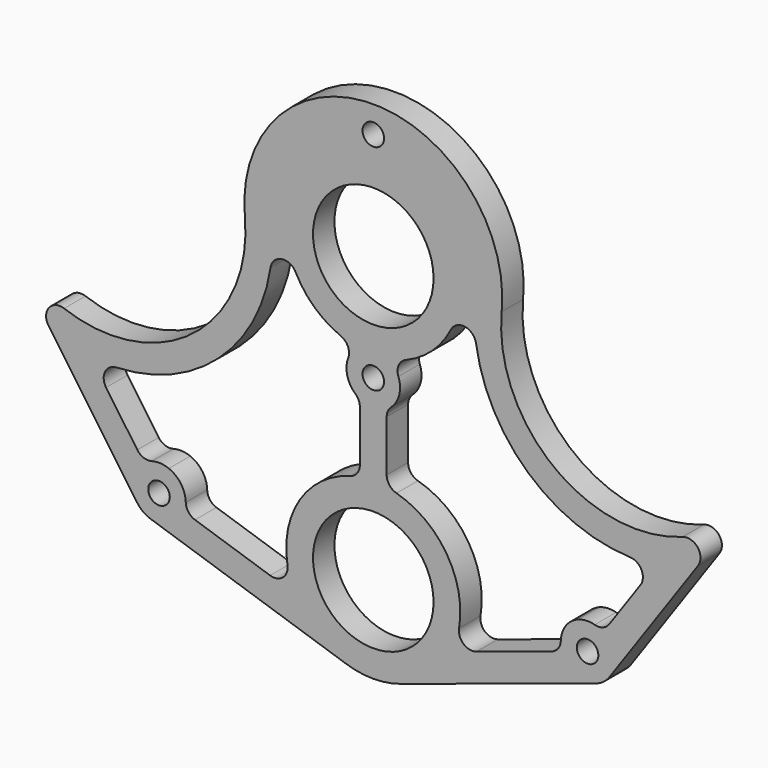
from build123d import *

# Parameters (mm, degrees)
F0_R     = 2.5527
F0_R_2   = 14.2875
F1_DEPTH = 6.35
F2_F1_R  = 3.175
F2_F2_R  = 3.175
F4_DEPTH = 25.4
F5_R     = 3.175


# Not quite as in the source:
# - a pattern or mirror of a feature is missing from the dataset's text; its kind, count and spacing are read off the source's solid


with BuildPart() as f1:
    # F0 (on Front) → F1 (new body)
    with BuildSketch(Plane.XZ):
        with BuildLine():
            ThreePointArc((-30.44415143, 64.2793510436), (-51.27863842, 31.2336995415), (-88.5449286211, 42.9518284873))
            Line((-88.5449286211, 42.9518284873), (-56.0059264265, -3.6360459351))
            ThreePointArc((-56.0059264265, -3.6360459351), (-54.5853345088, -5.0984058937), (-52.7745376605, -6.0352051355))
            Line((-52.7745376605, -6.0352051355), (-6.4172473966, -21.2019166903))
            ThreePointArc((-6.4172473966, -21.2019166903), (0, -22.225), (6.4172473966, -21.2019166903))
            Line((6.4172473966, -21.2019166903), (52.7745376605, -6.0352051355))
            ThreePointArc((52.7745376605, -6.0352051355), (54.5853345088, -5.0984058937), (56.0059264265, -3.6360459351))
            Line((56.0059264265, -3.6360459351), (88.5449286211, 42.9518284873))
            ThreePointArc((88.5449286211, 42.9518284873), (51.27863842, 31.2336995415), (30.44415143, 64.2793510436))
            ThreePointArc((30.44415143, 64.2793510436), (0, 97.7265), (-30.44415143, 64.2793510436))
        make_face()
        with Locations((-50.8, 0)):
            Circle(F0_R, mode=Mode.SUBTRACT)
        with Locations((0, -1.5875)):
            Circle(F0_R_2, mode=Mode.SUBTRACT)
        with Locations((50.8, 0)):
            Circle(F0_R, mode=Mode.SUBTRACT)
        with Locations((0, 40.5765)):
            Circle(F0_R, mode=Mode.SUBTRACT)
        with Locations((0, 65.9765)):
            Circle(F0_R_2, mode=Mode.SUBTRACT)
        with Locations((0, 91.3765)):
            Circle(F0_R, mode=Mode.SUBTRACT)
    extrude(amount=F1_DEPTH)

    # F2: fillet of radius 3.175 on 2 edges, made by hand

    # F2_f1
    f2_f1_edges = [f1.edges().sort_by_distance(p)[0] for p in [
        (-88.5449286211, -3.175, 42.9518284873),
    ]]
    fillet(f2_f1_edges, radius=F2_F1_R)

    # F2_f2
    f2_f2_edges = [f1.edges().sort_by_distance(p)[0] for p in [
        (88.5449286211, -3.175, 42.9518284873),
    ]]
    fillet(f2_f2_edges, radius=F2_F2_R)

    # F3 (on face) → F4 (cut)
    with BuildSketch(Plane.XZ.offset(6.35)):
        with BuildLine():
            Line((3.175, 35.0772394145), (3.175, 18.8043067186))
            ThreePointArc((3.175, 18.8043067186), (18.2678223179, 8.0142224503), (18.5965200171, -10.5360110216))
            Line((18.5965200171, -10.5360110216), (44.7647958403, -1.9745379709))
            ThreePointArc((44.7647958403, -1.9745379709), (45.0527871506, 2.7003757871), (48.4675934129, 5.9061293383))
            ThreePointArc((48.4675934129, 5.9061293383), (51.5398921213, 6.306746055), (54.4360459499, 5.2059254026))
            Line((54.4360459499, 5.2059254026), (67.0131976966, 23.2133234987))
            ThreePointArc((67.0131976966, 23.2133234987), (39.0870703991, 30.7510953733), (24.3679226321, 55.6515628324))
            ThreePointArc((24.3679226321, 55.6515628324), (21.7379294481, 58.3195031239), (18.3969634882, 56.6245942764))
            ThreePointArc((18.3969634882, 56.6245942764), (12.3594159846, 49.4492121774), (3.7699852595, 45.6862654673))
            ThreePointArc((3.7699852595, 45.6862654673), (6.3400365543, 40.2209321773), (3.175, 35.0772394145))
        make_face()
    f4 = extrude(amount=-F4_DEPTH, mode=Mode.SUBTRACT)

    # F4_copies: F4 across plane
    add(f4.mirror(Plane(origin=(0, 0, 0), x_dir=(0, 0, -1), z_dir=(-1, 0, 0))), mode=Mode.SUBTRACT)

    # F5
    f5_edges = [f1.edges().sort_by_distance(p)[0] for p in [
        (3.769985, -3.175, 45.686265),
        (3.175, -3.175, 35.077239),
        (3.175, -3.175, 18.804307),
        (18.59652, -3.175, -10.536011),
        (44.764796, -3.175, -1.974538),
        (54.436046, -3.175, 5.205925),
        (67.013198, -3.175, 23.213323),
        (-3.769985, -3.175, 45.686265),
        (-67.013198, -3.175, 23.213323),
        (-54.436046, -3.175, 5.205925),
        (-44.764796, -3.175, -1.974538),
        (-18.59652, -3.175, -10.536011),
        (-3.175, -3.175, 18.804307),
        (-3.175, -3.175, 35.077239),
    ]]
    fillet(f5_edges, radius=F5_R)


solid = f1.part
